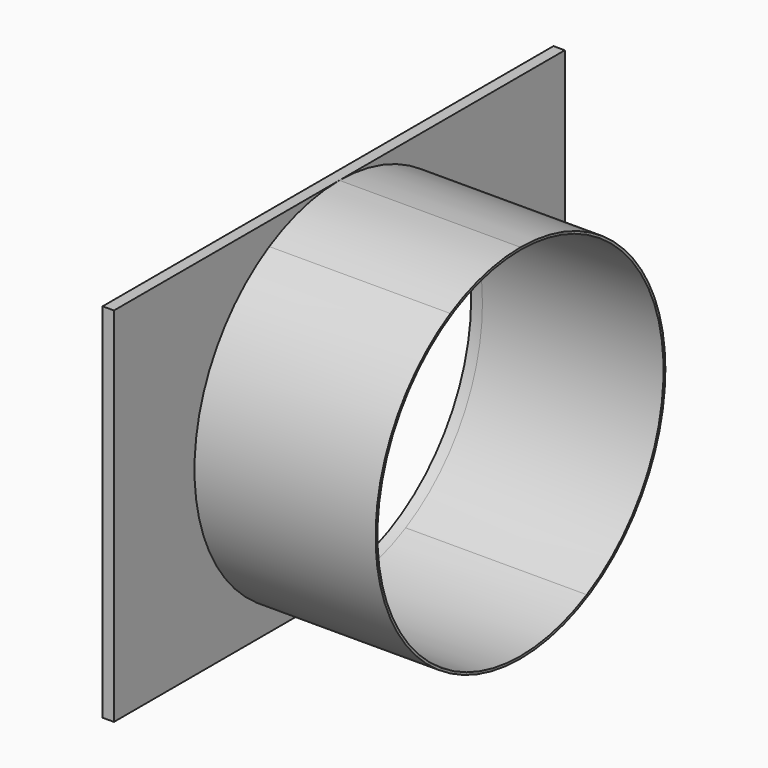
from build123d import *
from build123d import SkipClean  # not in build123d's __all__

# Parameters (mm, degrees)
F0_W     = 158.0642
F0_H     = 101.6
F0_R     = 50.165
F1_DEPTH = 3.175
F3_DEPTH = 50.8


with BuildPart() as f1:
    # F0 (on Right) → F1 (new body)
    with BuildSketch(Plane.YZ):
        Rectangle(F0_W, F0_H)
        Circle(F0_R, mode=Mode.SUBTRACT)
    extrude(amount=F1_DEPTH)

    # F2 (on face) → F3 (join)
    with BuildSketch(Plane.YZ.offset(3.175)):
        with BuildLine():
            Line((-23.253488448, 44.45), (-24.5934442484, 44.45))
            ThreePointArc((-24.5934442484, 44.45), (-50.8, 0), (-24.5934442484, -44.45))
            Line((-24.5934442484, -44.45), (-23.253488448, -44.45))
            ThreePointArc((-23.253488448, -44.45), (-50.165, 0), (-23.253488448, 44.45))
        make_face()
        with BuildLine():
            ThreePointArc((24.5934442484, -44.45), (43.7606385226, -25.8001262805), (50.8, 0))
            ThreePointArc((50.8, 0), (43.7606385226, 25.8001262805), (24.5934442484, 44.45))
            Line((24.5934442484, 44.45), (23.253488448, 44.45))
            ThreePointArc((23.253488448, 44.45), (42.9129262169, 25.9809158519), (50.165, 0))
            ThreePointArc((50.165, 0), (42.9129262169, -25.9809158519), (23.253488448, -44.45))
            Line((23.253488448, -44.45), (24.5934442484, -44.45))
        make_face()
        with BuildLine():
            Line((23.253488448, 44.45), (24.5934442484, 44.45))
            ThreePointArc((24.5934442484, 44.45), (12.6999999984, 49.1868884972), (-3.3e-09, 50.8))
            ThreePointArc((-3.3e-09, 50.8), (-12.7000000016, 49.1868884964), (-24.5934442484, 44.45))
            Line((-24.5934442484, 44.45), (-23.253488448, 44.45))
            ThreePointArc((-23.253488448, 44.45), (0, 50.165), (23.253488448, 44.45))
        make_face()
        with BuildLine():
            ThreePointArc((0, -50.8), (12.7, -49.1868884968), (24.5934442484, -44.45))
            Line((24.5934442484, -44.45), (23.253488448, -44.45))
            ThreePointArc((23.253488448, -44.45), (0, -50.165), (-23.253488448, -44.45))
            Line((-23.253488448, -44.45), (-24.5934442484, -44.45))
            ThreePointArc((-24.5934442484, -44.45), (-12.7, -49.1868884968), (0, -50.8))
        make_face()
    with SkipClean():  # cleaning this boolean's faces spoils the solid; the shape is the same uncleaned
        extrude(amount=F3_DEPTH)


solid = f1.part
